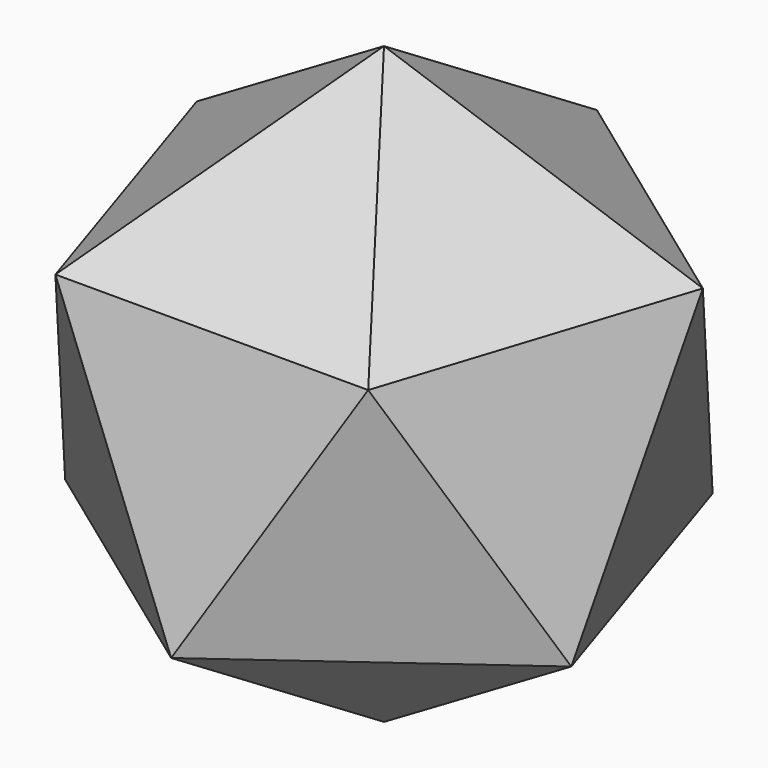
from build123d import *

# Parameters (mm, degrees)
F12_DEPTH      = 37.3243635206
F12_DEPTH_BACK = 37.3243635206
F15_DEPTH      = 37.3243635206
F15_DEPTH_BACK = 37.3243635206
F18_DEPTH      = 37.3243635206
F18_DEPTH_BACK = 37.3243635206
F21_DEPTH      = 37.3243635206
F21_DEPTH_BACK = 37.3243635206
F24_DEPTH      = 37.3243635206
F24_DEPTH_BACK = 37.3243635206
F28_DEPTH      = 99.1671965959
F28_DEPTH_BACK = 99.1671965959
F32_DEPTH      = 89.4601183415
F32_DEPTH_BACK = 89.4601183415
F35_DEPTH      = 89.4601183415
F35_DEPTH_BACK = 88.5596960493
F39_DEPTH      = 99.1671965959
F39_DEPTH_BACK = 96.8098604305
F42_DEPTH      = 68.0823305395
F42_DEPTH_BACK = 70.9961582856
F45_DEPTH      = 92.4043169267
F45_DEPTH_BACK = 99.1671965959
F48_DEPTH      = 81.4313769211
F48_DEPTH_BACK = 89.4601183415
F52_DEPTH      = 88.5596960493
F52_DEPTH_BACK = 82.3317992133
F56_DEPTH      = 92.4043169267
F56_DEPTH_BACK = 96.8098604305
F59_DEPTH      = 68.0823305395
F59_DEPTH_BACK = 68.0823305395
F62_DEPTH      = 37.3243635206
F62_DEPTH_BACK = 37.3243635206
F65_DEPTH      = 68.0823305395
F65_DEPTH_BACK = 68.0823305395
F68_DEPTH      = 81.4313769211
F68_DEPTH_BACK = 81.4313769211
F71_DEPTH      = 92.4043169267
F71_DEPTH_BACK = 92.4043169267
F74_DEPTH      = 92.4043169267
F74_DEPTH_BACK = 92.4043169267


# Not quite as in the source:
# - a feature names something its author has since deleted; it is built from what else it names


with BuildPart() as f9:
    # F7 (on Front) → F9 (revolve)
    with BuildSketch(Plane.XZ):
        with BuildLine():
            Line((0, 0), (0, 31.75))
            Line((0, 31.75), (0, 70.9951582856))
            ThreePointArc((0, 70.9951582856), (-70.9951582856, 0), (0, -70.9951582856))
            Line((0, -70.9951582856), (0, -31.75))
            Line((0, -31.75), (0, 0))
        make_face()
    revolve(axis=Axis((0, 0, -35.4975791428), (0, 0, -1)))

    # F11 (on 3pt) → F12 (cut, two sides)
    with BuildSketch(Plane(origin=(0, 0, 0), x_dir=(-0.5877852523, 0.8090169944, 0), z_dir=(0.8090169944, 0.5877852523, 0))) as f12_sk:
        Polygon((-63.5, -70.9951582856), (0, -70.9951582856), (-51.3725791428, -31.75), (-63.5, -31.75), align=None)
    extrude(amount=F12_DEPTH, mode=Mode.SUBTRACT)
    extrude(f12_sk.sketch, amount=-F12_DEPTH_BACK, mode=Mode.SUBTRACT)

    # F14 (on 3pt) → F15 (cut, two sides)
    with BuildSketch(Plane(origin=(0, 0, 0), x_dir=(-0.5877852523, -0.8090169944, 0), z_dir=(-0.8090169944, 0.5877852523, 0))) as f15_sk:
        Polygon((51.3725791428, -31.75), (0, -70.9951582856), (63.5, -70.9951582856), (63.5, -31.75), align=None)
    extrude(amount=-F15_DEPTH, mode=Mode.SUBTRACT)
    extrude(f15_sk.sketch, amount=F15_DEPTH_BACK, mode=Mode.SUBTRACT)

    # F17 (on 3pt) → F18 (cut, two sides)
    with BuildSketch(Plane(origin=(0, 0, 0), x_dir=(0.9510565163, -0.3090169944, 0), z_dir=(-0.3090169944, -0.9510565163, 0))) as f18_sk:
        Polygon((-63.5, -70.9951582856), (0, -70.9951582856), (-51.3725791428, -31.75), (-63.5, -31.75), align=None)
    extrude(amount=-F18_DEPTH, mode=Mode.SUBTRACT)
    extrude(f18_sk.sketch, amount=F18_DEPTH_BACK, mode=Mode.SUBTRACT)

    # F20 (on 3pt) → F21 (cut, two sides)
    with BuildSketch(Plane.YZ) as f21_sk:
        Polygon((51.3725791428, -31.75), (0, -70.9951582856), (63.5, -70.9951582856), (63.5, -31.75), align=None)
    extrude(amount=-F21_DEPTH, mode=Mode.SUBTRACT)
    extrude(f21_sk.sketch, amount=F21_DEPTH_BACK, mode=Mode.SUBTRACT)

    # F23 (on 3pt) → F24 (cut, two sides)
    with BuildSketch(Plane(origin=(0, 0, 0), x_dir=(-0.9510565163, -0.3090169944, 0), z_dir=(-0.3090169944, 0.9510565163, 0))) as f24_sk:
        Polygon((-63.5, -70.9951582856), (0, -70.9951582856), (-51.3725791428, -31.75), (-63.5, -31.75), align=None)
    extrude(amount=F24_DEPTH, mode=Mode.SUBTRACT)
    extrude(f24_sk.sketch, amount=-F24_DEPTH_BACK, mode=Mode.SUBTRACT)

    # F27 (on 3pt) → F28 (cut, two sides)
    with BuildSketch(Plane(origin=(0, 0, 0), x_dir=(-0.5877852523, 0.8090169944, 0), z_dir=(0.8090169944, 0.5877852523, 0))) as f28_sk:
        Polygon((-70.9951582856, -31.75), (-51.3725791428, -31.75), (-63.5, 31.75), (-70.9951582856, 31.75), align=None)
    extrude(amount=F28_DEPTH, mode=Mode.SUBTRACT)
    extrude(f28_sk.sketch, amount=-F28_DEPTH_BACK, mode=Mode.SUBTRACT)

    # F31 (on 3pt) → F32 (cut, two sides)
    with BuildSketch(Plane(origin=(0, 0, 0), x_dir=(0.9510565163, -0.3090169944, 0), z_dir=(-0.3090169944, -0.9510565163, 0))) as f32_sk:
        Polygon((70.9951582856, 31.75), (51.3725791428, 31.75), (63.5, -31.75), (70.9951582856, -31.75), align=None)
    extrude(amount=-F32_DEPTH, mode=Mode.SUBTRACT)
    extrude(f32_sk.sketch, amount=F32_DEPTH_BACK, mode=Mode.SUBTRACT)

    # F34 (on 3pt) → F35 (cut, two sides)
    with BuildSketch(Plane(origin=(0, 0, 0), x_dir=(0.9510565163, 0.3090169944, 0), z_dir=(0.3090169944, -0.9510565163, 0))) as f35_sk:
        Polygon((63.5, 31.75), (51.3725791428, -31.75), (70.9951582856, -31.75), (70.9951582856, 31.75), align=None)
    extrude(amount=-F35_DEPTH, mode=Mode.SUBTRACT)
    extrude(f35_sk.sketch, amount=F35_DEPTH_BACK, mode=Mode.SUBTRACT)

    # F38 (on 3pt) → F39 (cut, two sides)
    with BuildSketch(Plane(origin=(0, 0, 0), x_dir=(0.5877852523, 0.8090169944, 0), z_dir=(0.8090169944, -0.5877852523, 0))) as f39_sk:
        Polygon((70.9951582856, 31.75), (51.3725791428, 31.75), (63.5, -31.75), (70.9951582856, -31.75), align=None)
    extrude(amount=-F39_DEPTH, mode=Mode.SUBTRACT)
    extrude(f39_sk.sketch, amount=F39_DEPTH_BACK, mode=Mode.SUBTRACT)

    # F41 (on 3pt) → F42 (cut, two sides)
    with BuildSketch(Plane(origin=(0, 0, 0), x_dir=(0, -1, 0), z_dir=(-1, 0, 0))) as f42_sk:
        Polygon((-70.9951582856, -31.75), (-51.3725791428, -31.75), (-63.5, 31.75), (-70.9951582856, 31.75), align=None)
    extrude(amount=-F42_DEPTH, mode=Mode.SUBTRACT)
    extrude(f42_sk.sketch, amount=F42_DEPTH_BACK, mode=Mode.SUBTRACT)

    # F44 (on 3pt) → F45 (cut, two sides)
    with BuildSketch(Plane(origin=(0, 0, 0), x_dir=(0.5877852523, -0.8090169944, 0), z_dir=(-0.8090169944, -0.5877852523, 0))) as f45_sk:
        Polygon((-63.5, -31.75), (-51.3725791428, 31.75), (-70.9951582856, 31.75), (-70.9951582856, -31.75), align=None)
    extrude(amount=-F45_DEPTH, mode=Mode.SUBTRACT)
    extrude(f45_sk.sketch, amount=F45_DEPTH_BACK, mode=Mode.SUBTRACT)

    # F47 (on 3pt) → F48 (cut, two sides)
    with BuildSketch(Plane(origin=(0, 0, 0), x_dir=(0.9510565163, -0.3090169944, 0), z_dir=(-0.3090169944, -0.9510565163, 0))) as f48_sk:
        Polygon((-70.9951582856, -31.75), (-51.3725791428, -31.75), (-63.5, 31.75), (-70.9951582856, 31.75), align=None)
    extrude(amount=-F48_DEPTH, mode=Mode.SUBTRACT)
    extrude(f48_sk.sketch, amount=F48_DEPTH_BACK, mode=Mode.SUBTRACT)

    # F51 (on 3pt) → F52 (cut, two sides)
    with BuildSketch(Plane(origin=(0, 0, 0), x_dir=(-0.9510565163, -0.3090169944, 0), z_dir=(-0.3090169944, 0.9510565163, 0))) as f52_sk:
        Polygon((70.9951582856, 31.75), (51.3725791428, 31.75), (63.5, -31.75), (70.9951582856, -31.75), align=None)
    extrude(amount=-F52_DEPTH, mode=Mode.SUBTRACT)
    extrude(f52_sk.sketch, amount=F52_DEPTH_BACK, mode=Mode.SUBTRACT)

    # F55 (on 3pt) → F56 (cut, two sides)
    with BuildSketch(Plane(origin=(0, 0, 0), x_dir=(0.5877852523, 0.8090169944, 0), z_dir=(0.8090169944, -0.5877852523, 0))) as f56_sk:
        Polygon((-70.9951582856, -31.75), (-51.3725791428, -31.75), (-63.5, 31.75), (-70.9951582856, 31.75), align=None)
    extrude(amount=-F56_DEPTH, mode=Mode.SUBTRACT)
    extrude(f56_sk.sketch, amount=F56_DEPTH_BACK, mode=Mode.SUBTRACT)

    # F58 (on 3pt) → F59 (cut, two sides)
    with BuildSketch(Plane(origin=(0, 0, 0), x_dir=(0, -1, 0), z_dir=(-1, 0, 0))) as f59_sk:
        Polygon((70.9951582856, 31.75), (51.3725791428, 31.75), (63.5, -31.75), (70.9951582856, -31.75), align=None)
    extrude(amount=-F59_DEPTH, mode=Mode.SUBTRACT)
    extrude(f59_sk.sketch, amount=F59_DEPTH_BACK, mode=Mode.SUBTRACT)

    # F61 (on 3pt) → F62 (cut, two sides)
    with BuildSketch(Plane(origin=(0, 0, 0), x_dir=(0.9510565163, -0.3090169944, 0), z_dir=(-0.3090169944, -0.9510565163, 0))) as f62_sk:
        Polygon((63.5, 70.9951582856), (0, 70.9951582856), (51.3725791428, 31.75), (63.5, 31.75), align=None)
    extrude(amount=F62_DEPTH, mode=Mode.SUBTRACT)
    extrude(f62_sk.sketch, amount=-F62_DEPTH_BACK, mode=Mode.SUBTRACT)

    # F64 (on 3pt) → F65 (cut, two sides)
    with BuildSketch(Plane.YZ) as f65_sk:
        Polygon((-51.3725791428, 31.75), (0, 70.9951582856), (-63.5, 70.9951582856), (-63.5, 31.75), align=None)
    extrude(amount=-F65_DEPTH, mode=Mode.SUBTRACT)
    extrude(f65_sk.sketch, amount=F65_DEPTH_BACK, mode=Mode.SUBTRACT)

    # F67 (on 3pt) → F68 (cut, two sides)
    with BuildSketch(Plane(origin=(0, 0, 0), x_dir=(0.9510565163, 0.3090169944, 0), z_dir=(0.3090169944, -0.9510565163, 0))) as f68_sk:
        Polygon((-51.3725791428, 31.75), (0, 70.9951582856), (-63.5, 70.9951582856), (-63.5, 31.75), align=None)
    extrude(amount=-F68_DEPTH, mode=Mode.SUBTRACT)
    extrude(f68_sk.sketch, amount=F68_DEPTH_BACK, mode=Mode.SUBTRACT)

    # F70 (on 3pt) → F71 (cut, two sides)
    with BuildSketch(Plane(origin=(0, 0, 0), x_dir=(-0.5877852523, 0.8090169944, 0), z_dir=(0.8090169944, 0.5877852523, 0))) as f71_sk:
        Polygon((63.5, 70.9951582856), (0, 70.9951582856), (51.3725791428, 31.75), (63.5, 31.75), align=None)
    extrude(amount=-F71_DEPTH, mode=Mode.SUBTRACT)
    extrude(f71_sk.sketch, amount=F71_DEPTH_BACK, mode=Mode.SUBTRACT)

    # F73 (on 3pt) → F74 (cut, two sides)
    with BuildSketch(Plane(origin=(0, 0, 0), x_dir=(0.5877852523, 0.8090169944, 0), z_dir=(0.8090169944, -0.5877852523, 0))) as f74_sk:
        Polygon((63.5, 70.9951582856), (0, 70.9951582856), (51.3725791428, 31.75), (63.5, 31.75), align=None)
    extrude(amount=-F74_DEPTH, mode=Mode.SUBTRACT)
    extrude(f74_sk.sketch, amount=F74_DEPTH_BACK, mode=Mode.SUBTRACT)


solid = f9.part
